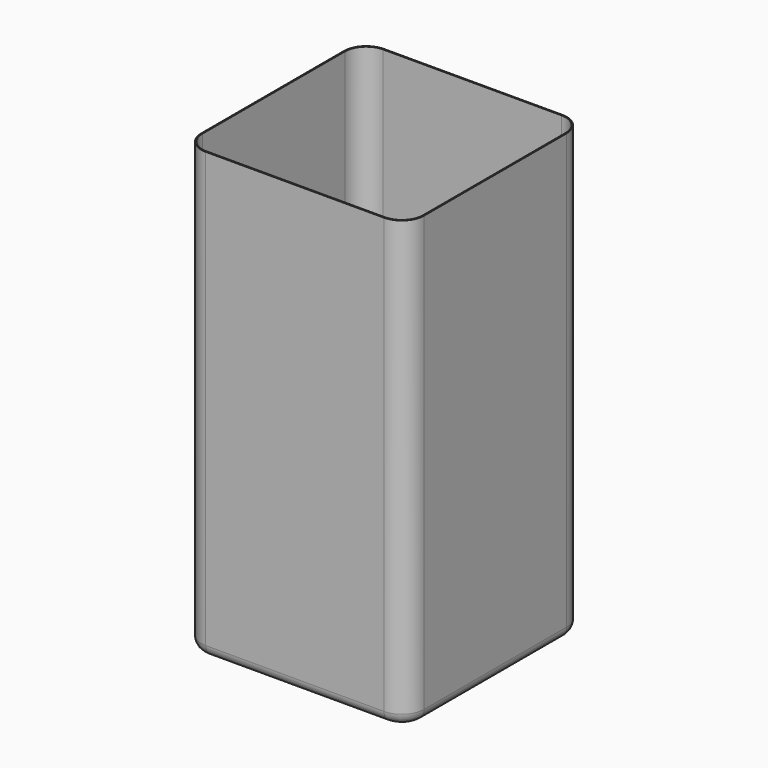
from build123d import *

# Parameters (mm, degrees)
F1_DEPTH     = 1016
F2_R         = 25.4
F3_T1_DEPTH  = 1143
F3_T4_ANGLE  = 90
F3_T6_ANGLE  = 90
F3_T8_ANGLE  = 90
F3_T10_ANGLE = 90
F4_T         = -2.54


# Not quite as in the source:
# - a fillet or chamfer that OpenCascade refuses, or shapes differently, is made with other operations: its cross-section is extruded or revolved along the edge and cut away or added


with BuildPart() as f1:
    # F0 (on Top) → F1 (new body)
    with BuildSketch(Plane.XY):
        Polygon((254, -254), (254, 0), (254, 254), (-254, 254), (-254, -254), align=None)
    extrude(amount=F1_DEPTH)

    # F2
    f2_edges = [f1.edges().sort_by_distance(p)[0] for p in [
        (-254, 0, 0),
        (0, 254, 0),
        (0, -254, 0),
        (254, 0, 0),
    ]]
    fillet(f2_edges, radius=F2_R)

    # F3: fillet of radius 50.8 on 4 edges, made by hand

    # F3_s2 → F3_t1 (cut)
    with BuildSketch(Plane.XY):
        with BuildLine():
            ThreePointArc((-203.2, 254), (-239.1210244843, 239.1210244843), (-254, 203.2))
            Line((-254, 203.2), (-254, 254))
            Line((-254, 254), (-203.2, 254))
        make_face()
        with BuildLine():
            ThreePointArc((-203.2, -254), (-239.1210244843, -239.1210244843), (-254, -203.2))
            Line((-254, -203.2), (-254, -254))
            Line((-254, -254), (-203.2, -254))
        make_face()
        with BuildLine():
            ThreePointArc((254, 203.2), (239.1210244843, 239.1210244843), (203.2, 254))
            Line((203.2, 254), (254, 254))
            Line((254, 254), (254, 203.2))
        make_face()
        with BuildLine():
            ThreePointArc((254, -203.2), (239.1210244843, -239.1210244843), (203.2, -254))
            Line((203.2, -254), (254, -254))
            Line((254, -254), (254, -203.2))
        make_face()
    extrude(amount=F3_T1_DEPTH, mode=Mode.SUBTRACT)

    # F3_s3 → F3_t4 (revolve, cut)
    with BuildSketch(Plane.XZ.offset(203.2)):
        with BuildLine():
            ThreePointArc((228.6, 0), (246.5605122421, 7.4394877579), (254, 25.4))
            Line((254, 25.4), (254, 0))
            Line((254, 0), (228.6, 0))
        make_face()
    revolve(axis=Axis((203.2, -203.2, 0), (0, 0, -1)), revolution_arc=F3_T4_ANGLE, mode=Mode.SUBTRACT)

    # F3_s5 → F3_t6 (revolve, cut)
    with BuildSketch(Plane.YZ.offset(203.2)):
        with BuildLine():
            ThreePointArc((228.6, 0), (246.5605122421, 7.4394877579), (254, 25.4))
            Line((254, 25.4), (254, 0))
            Line((254, 0), (228.6, 0))
        make_face()
    revolve(axis=Axis((203.2, 203.2, 0), (0, 0, -1)), revolution_arc=F3_T6_ANGLE, mode=Mode.SUBTRACT)

    # F3_s7 → F3_t8 (revolve, cut)
    with BuildSketch(Plane.YZ.offset(-203.2)):
        with BuildLine():
            ThreePointArc((-228.6, 0), (-246.5605122421, 7.4394877579), (-254, 25.4))
            Line((-254, 25.4), (-254, 0))
            Line((-254, 0), (-228.6, 0))
        make_face()
    revolve(axis=Axis((-203.2, -203.2, 0), (0, 0, -1)), revolution_arc=F3_T8_ANGLE, mode=Mode.SUBTRACT)

    # F3_s9 → F3_t10 (revolve, cut)
    with BuildSketch(Plane.XZ.offset(-203.2)):
        with BuildLine():
            ThreePointArc((-228.6, 0), (-246.5605122421, 7.4394877579), (-254, 25.4))
            Line((-254, 25.4), (-254, 0))
            Line((-254, 0), (-228.6, 0))
        make_face()
    revolve(axis=Axis((-203.2, 203.2, 0), (0, 0, -1)), revolution_arc=F3_T10_ANGLE, mode=Mode.SUBTRACT)

    # F4
    f4_openings = [f1.faces().sort_by_distance(p)[0] for p in [
        (0, 0, 1016),
    ]]
    offset(amount=F4_T, openings=f4_openings)


solid = f1.part
